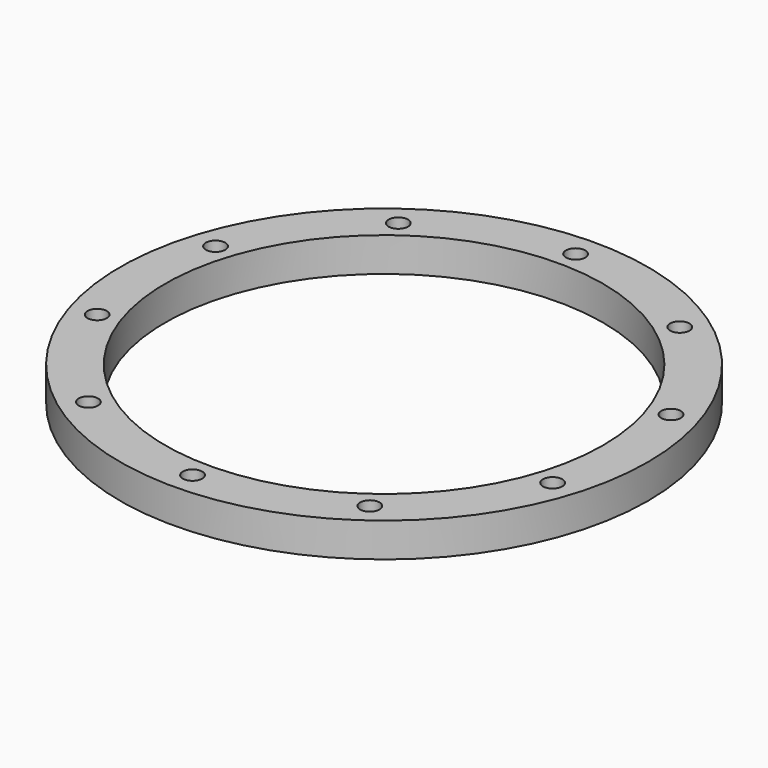
from build123d import *

# Parameters (mm, degrees)
F0_R            = 115.75
F0_R_2          = 96
F1_DEPTH        = 15
F3_D            = 8.5
F3_COPIES_COUNT = 10


# Not quite as in the source:
# - a pattern or mirror of a feature is missing from the dataset's text; its kind, count and spacing are read off the source's solid


with BuildPart() as f1:
    # F0 (on Top) → F1 (new body)
    with BuildSketch(Plane.XY):
        Circle(F0_R)
        Circle(F0_R_2, mode=Mode.SUBTRACT)
    extrude(amount=F1_DEPTH)

    # F3 (through all)
    with Locations(Plane.XY.offset(15)):
        with Locations((0, 105)):
            f3 = Hole(F3_D / 2)

    # F3_copies: F3 ×10 about axis
    f3_copies_axis = Axis((0, 0, 0), (0, 0, 1))
    for i in range(1, F3_COPIES_COUNT):
        add(f3.rotate(f3_copies_axis, i * 360 / F3_COPIES_COUNT), mode=Mode.SUBTRACT)


solid = f1.part
